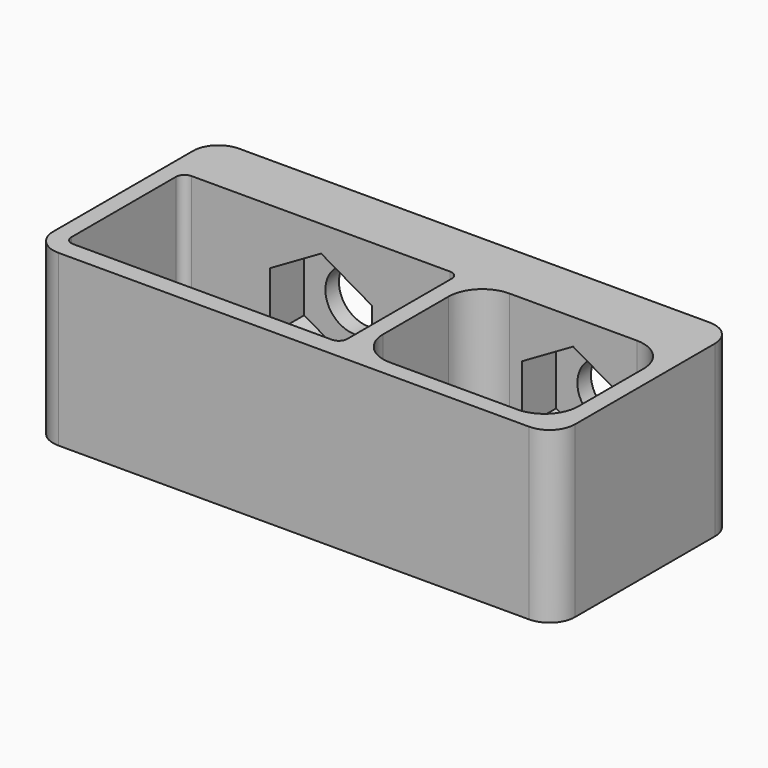
from build123d import *

# Parameters (mm, degrees)
F0_W     = 30.75
F0_H     = 13.3
F0_W_2   = 16.25
F0_H_2   = 8.7
F0_W_3   = 11.5
F0_H_3   = 8.8
F1_DEPTH = 10
F2_R     = 0.5
F3_R     = 2
F4_R     = 1.5
F7_DEPTH = 2.5
F5_R     = 1.75
F8_DEPTH = 8


with BuildPart() as f1:
    # F0 (on Top) → F1 (new body)
    with BuildSketch(Plane.XY):
        with Locations((-14.5149128214, -8.8939947993)):
            Rectangle(F0_W, F0_H)
        with Locations((-20.7649128214, -10.0939947993)):
            Rectangle(F0_W_2, F0_H_2, mode=Mode.SUBTRACT)
        with Locations((-5.8899128214, -10.1439947993)):
            Rectangle(F0_W_3, F0_H_3, mode=Mode.SUBTRACT)
    extrude(amount=F1_DEPTH)

    # F2
    f2_edges = [f1.edges().sort_by_distance(p)[0] for p in [
        (-28.889913, -5.743995, 5),
        (-28.889913, -14.443995, 5),
        (-12.639913, -5.743995, 5),
        (-12.639913, -14.443995, 5),
    ]]
    fillet(f2_edges, radius=F2_R)

    # F3
    f3_edges = [f1.edges().sort_by_distance(p)[0] for p in [
        (-0.139913, -5.743995, 5),
        (-0.139913, -14.543995, 5),
        (-11.639913, -14.543995, 5),
        (-11.639913, -5.743995, 5),
    ]]
    fillet(f3_edges, radius=F3_R)

    # F4
    f4_edges = [f1.edges().sort_by_distance(p)[0] for p in [
        (-29.889913, -15.543995, 5),
        (-29.889913, -2.243995, 5),
        (0.860087, -15.543995, 5),
        (0.860087, -2.243995, 5),
    ]]
    fillet(f4_edges, radius=F4_R)

    # F6 (on face) → F7 (cut)
    with BuildSketch(Plane.XZ.offset(5.7439947993)):
        Polygon((-8.8899128214, 6.7320508076), (-8.8899128214, 3.2679491924), (-5.8899128214, 1.5358983849), (-2.8899128214, 3.2679491924), (-2.8899128214, 6.7320508076), (-5.8899128214, 8.4641016151), align=None)
        Polygon((-23.7399128214, 6.7320508076), (-23.7399128214, 3.2679491924), (-20.7399128214, 1.5358983849), (-17.7399128214, 3.2679491924), (-17.7399128214, 6.7320508076), (-20.7399128214, 8.4641016151), align=None)
    extrude(amount=-F7_DEPTH, mode=Mode.SUBTRACT)

    # F5 (on face) → F8 (cut)
    with BuildSketch(Plane(origin=(0, -2.2439947993, 0), x_dir=(-1, 0, 0), z_dir=(0, 1, 0))):
        with Locations((5.8899128214, 5)):
            Circle(F5_R)
        with Locations((20.7399128214, 5)):
            Circle(F5_R)
    extrude(amount=-F8_DEPTH, mode=Mode.SUBTRACT)


solid = f1.part
